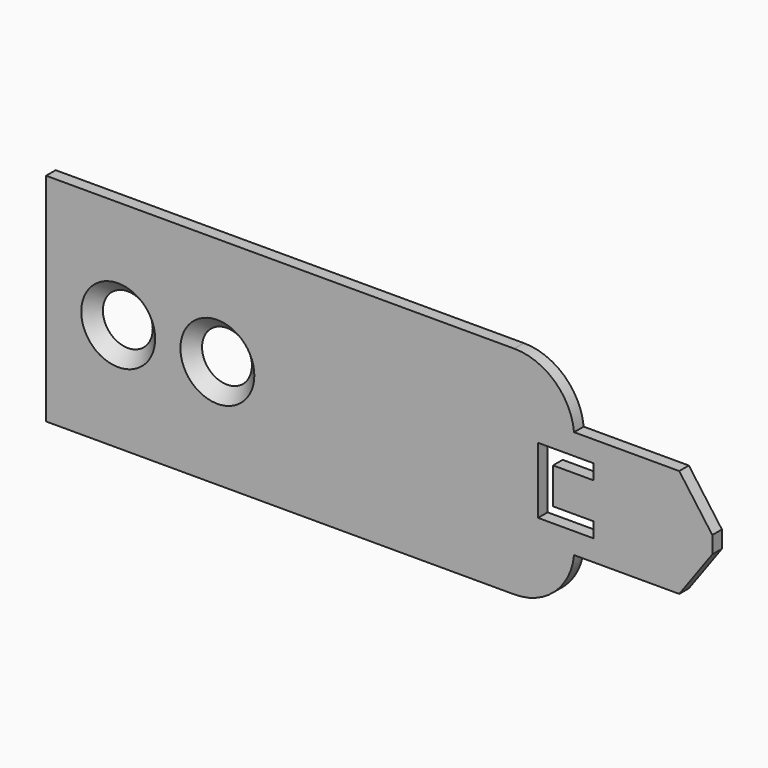
from build123d import *

# Parameters (mm, degrees)
F0_R        = 4.15
F1_DEPTH    = 2
F2_SIZE     = 1.99999
F3_T1_DEPTH = 51.7493718553


# Not quite as in the source:
# - a fillet or chamfer that OpenCascade refuses, or shapes differently, is made with other operations: its cross-section is extruded or revolved along the edge and cut away or added
# - a fillet or chamfer is up to 0.001 mm smaller than in the source, because OpenCascade refuses the exact size


with BuildPart() as f1:
    # F0 (on Front) → F1 (new body)
    with BuildSketch(Plane.XZ):
        Polygon((87.85, 18), (0, 18), (0, -18), (87.85, -18), (87.85, -9), (105.35, -9), (110.85, -1.42), (110.85, 1.42), (105.35, 9), (87.85, 9), align=None)
        with Locations((12, 0)):
            Circle(F0_R, mode=Mode.SUBTRACT)
        with Locations((28.5, 0)):
            Circle(F0_R, mode=Mode.SUBTRACT)
        Polygon((91.1, 5.5), (91.1, 3), (84.35, 3), (84.35, -3), (91.1, -3), (91.1, -5.5), (81.85, -5.5), (81.85, 5.5), align=None, mode=Mode.SUBTRACT)
    extrude(amount=F1_DEPTH)

    # F2 (size 2 in the source; OpenCascade refuses exactly that, so slightly less here)
    f2_edges = [f1.edges().sort_by_distance(p)[0] for p in [
        (7.85, -2, 0),
        (24.35, -2, 0),
    ]]
    chamfer(f2_edges, length=F2_SIZE)

    # F3: fillet of radius 10 on 2 edges, made by hand

    # F3_s2 → F3_t1 (cut)
    with BuildSketch(Plane.XZ.offset(-24.8746859277)):
        with BuildLine():
            ThreePointArc((77.9001256289, 18), (84.6083295614, 15.4161984871), (87.85, 9))
            Line((87.85, 9), (87.85, 18))
            Line((87.85, 18), (77.9001256289, 18))
        make_face()
        with BuildLine():
            ThreePointArc((77.9001256289, -18), (84.6083295614, -15.4161984871), (87.85, -9))
            Line((87.85, -9), (87.85, -18))
            Line((87.85, -18), (77.9001256289, -18))
        make_face()
    extrude(amount=F3_T1_DEPTH, mode=Mode.SUBTRACT)


solid = f1.part
